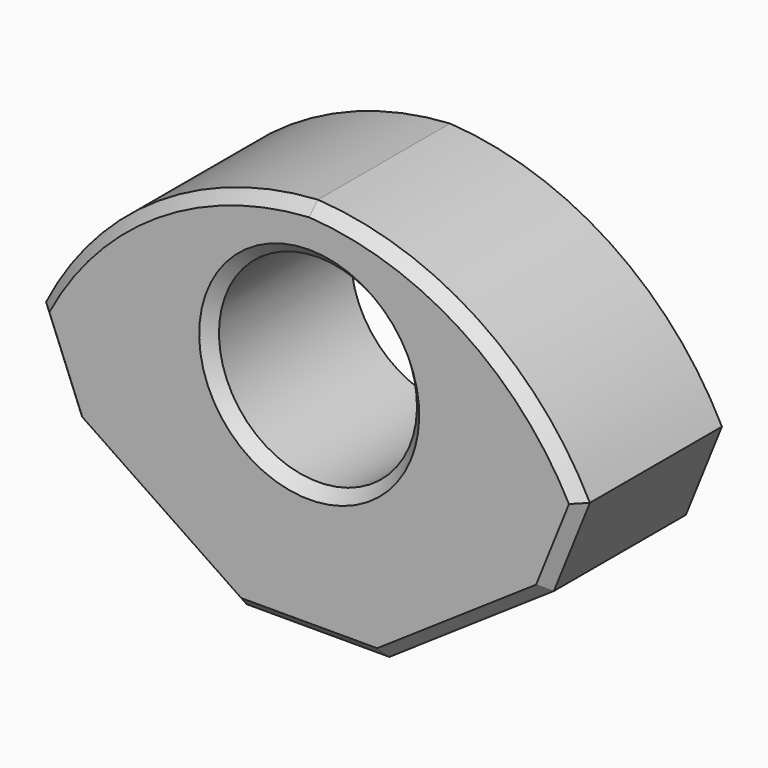
from build123d import *

# Parameters (mm, degrees)
F1_DEPTH   = 80
F2_C1_SIZE = 5
F2_C2_SIZE = 5
F2_C3_SIZE = 5
F2_C4_SIZE = 5
F2_C5_SIZE = 5
F2_C6_SIZE = 5
F2_C7_SIZE = 5
F2_C8_SIZE = 5


with BuildPart() as f1:
    # F0 (on Front) → F1 (new body)
    with BuildSketch(Plane.XZ):
        with BuildLine():
            Line((0, 58.1298414463), (0, 81.0960731047))
            ThreePointArc((0, 81.0960731047), (-72.594350102, 57.0156445727), (-123.5749638583, 0))
            Line((-123.5749638583, 0), (-107.2012897506, -40.625271212))
            Line((-107.2012897506, -40.625271212), (-32.4384310855, -91.2910051649))
            Line((-32.4384310855, -91.2910051649), (0, -91.2910051649))
            Line((0, -91.2910051649), (0, -31.8701585537))
            ThreePointArc((0, -31.8701585537), (-45, 13.1298414463), (0, 58.1298414463))
        make_face()
        with BuildLine():
            ThreePointArc((123.5749638583, 0), (72.594350102, 57.0156445727), (0, 81.0960731047))
            Line((0, 81.0960731047), (0, 58.1298414463))
            ThreePointArc((0, 58.1298414463), (31.8198051534, 44.9496465997), (45, 13.1298414463))
            ThreePointArc((45, 13.1298414463), (31.8198051534, -18.6899637071), (0, -31.8701585537))
            Line((0, -31.8701585537), (0, -91.2910051649))
            Line((0, -91.2910051649), (32.4384310855, -91.2910051649))
            Line((32.4384310855, -91.2910051649), (107.2012897506, -40.625271212))
            Line((107.2012897506, -40.625271212), (123.5749638583, 0))
        make_face()
    extrude(amount=F1_DEPTH)

    # F2: chamfer of 5 on 8 edges, made by hand

    # F2_c1
    f2_c1_edges = [f1.edges().sort_by_distance(p)[0] for p in [
        (0, -80, -31.8701585537),
    ]]
    chamfer(f2_c1_edges, length=F2_C1_SIZE)

    # F2_c2
    f2_c2_edges = [f1.edges().sort_by_distance(p)[0] for p in [
        (-72.594350102, -80, 57.0156445727),
    ]]
    chamfer(f2_c2_edges, length=F2_C2_SIZE)

    # F2_c3
    f2_c3_edges = [f1.edges().sort_by_distance(p)[0] for p in [
        (-114.129610425, -80, -23.4351827451),
    ]]
    chamfer(f2_c3_edges, length=F2_C3_SIZE)

    # F2_c4
    f2_c4_edges = [f1.edges().sort_by_distance(p)[0] for p in [
        (-66.1115818198, -80, -68.4711862478),
    ]]
    chamfer(f2_c4_edges, length=F2_C4_SIZE)

    # F2_c5
    f2_c5_edges = [f1.edges().sort_by_distance(p)[0] for p in [
        (4.4563329797, -80, -91.2910051649),
    ]]
    chamfer(f2_c5_edges, length=F2_C5_SIZE)

    # F2_c6
    f2_c6_edges = [f1.edges().sort_by_distance(p)[0] for p in [
        (73.5088851707, -80, -63.4581381884),
    ]]
    chamfer(f2_c6_edges, length=F2_C6_SIZE)

    # F2_c7
    f2_c7_edges = [f1.edges().sort_by_distance(p)[0] for p in [
        (117.0626938618, -80, -16.1578111957),
    ]]
    chamfer(f2_c7_edges, length=F2_C7_SIZE)

    # F2_c8
    f2_c8_edges = [f1.edges().sort_by_distance(p)[0] for p in [
        (86.848352424, -80, 46.3883216842),
    ]]
    chamfer(f2_c8_edges, length=F2_C8_SIZE)


solid = f1.part
